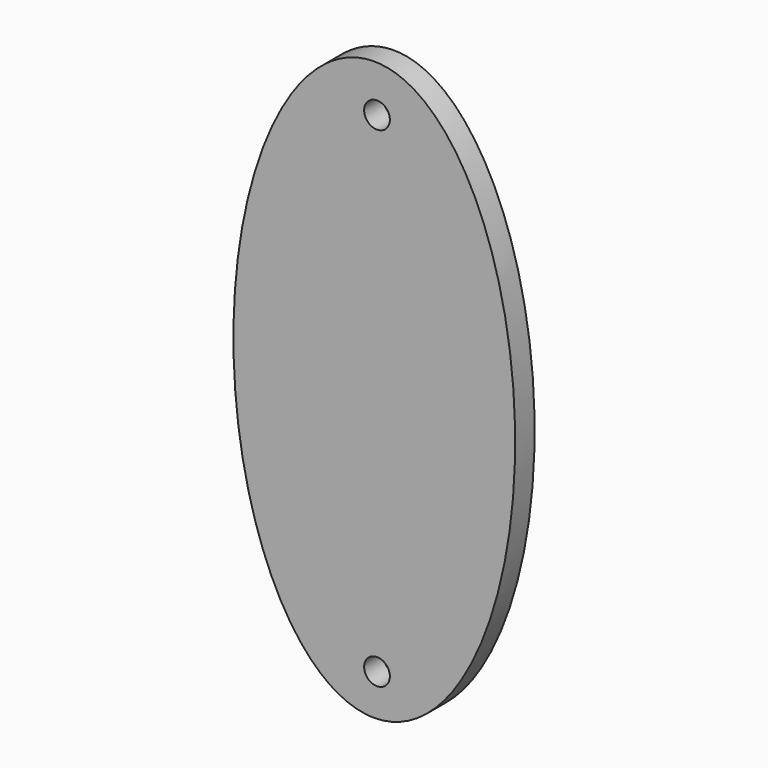
from build123d import *

# Parameters (mm, degrees)
F1_DEPTH = 5
F2_R     = 2.6459382912
F3_DEPTH = 25


# Not quite as in the source:
# - a feature names something its author has since deleted; it is built from what else it names


with BuildPart() as f1:
    # F0 (on Front) → F1 (new body)
    with BuildSketch(Plane.XZ):
        with BuildLine():
            add(Edge.make_bspline(
                [(18.7854766846, -23.277670145), (68.9568782657, -23.277670145), (43.8711774751, 65.8513084054), (18.7854766846, 154.9802869558), (-6.300224106, 65.8513084054), (-31.3859248966, -23.277670145), (18.7854766846, -23.277670145)],
                knots=[0, 0, 0, 2.0943951024, 2.0943951024, 4.1887902048, 4.1887902048, 6.2831853072, 6.2831853072, 6.2831853072], degree=2, weights=[1, 0.5, 1, 0.5, 1, 0.5, 1]))
        make_face()
    extrude(amount=F1_DEPTH)

    # F2 (on face) → F3 (cut)
    with BuildSketch(Plane.XZ):
        with Locations((19.3407479674, 86.0370546579)):
            Circle(F2_R)
        with Locations((19.3407479674, -14.7185996175)):
            Circle(F2_R)
    extrude(amount=F3_DEPTH, mode=Mode.SUBTRACT)


solid = f1.part
